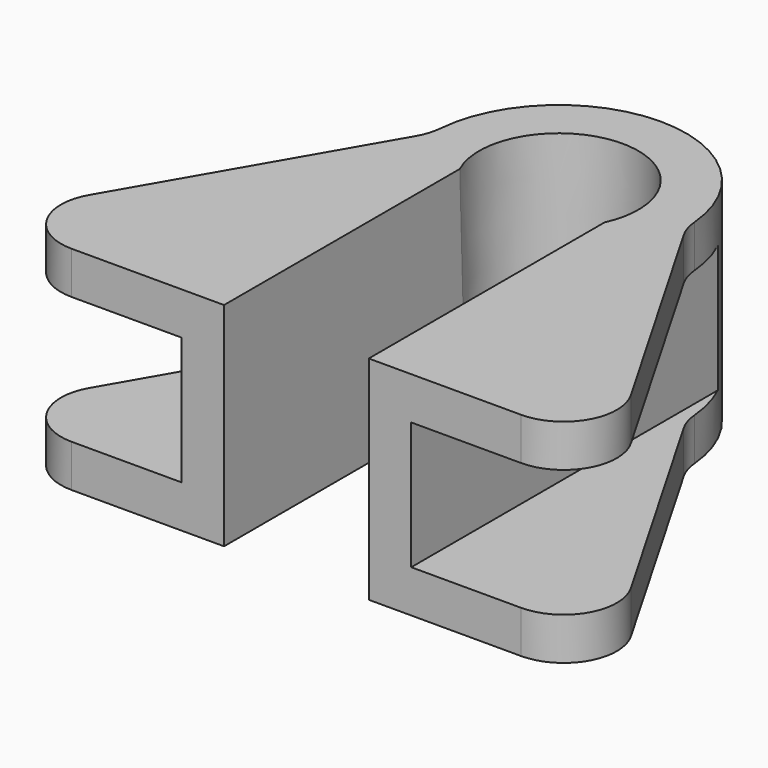
from build123d import *

# Parameters (mm, degrees)
F3_R      = 24
F4_DEPTH  = 40
F0_R      = 15
F2_R      = 14.5
F7_DEPTH  = 40.0010001
F9_DEPTH  = 40
F10_W     = 38.0299583572
F10_H     = 24
F11_DEPTH = 85.7581399225
F12_R     = 10
F13_R     = 10


# Not quite as in the source:
# - a pattern or mirror of a feature is missing from the dataset's text; its kind, count and spacing are read off the source's solid


with BuildPart() as f4:
    # F3 (on Top) → F4 (new body)
    with BuildSketch(Plane.XY):
        Circle(F3_R)
    extrude(amount=-F4_DEPTH)

    # F0 (on Top) → F5 section 0
    with BuildSketch(Plane.XY):
        Circle(F0_R)
    # F2 (on offset) → F5 section 1
    with BuildSketch(Plane.XY.offset(-40)):
        Circle(F2_R)
    loft(mode=Mode.SUBTRACT)

    # F6 (on face) → F7 (cut, through all)
    with BuildSketch(Plane.XY):
        with BuildLine():
            Line((-13.6255430014, -6.272525641), (-13.6255430014, -19.7571399225))
            ThreePointArc((-13.6255430014, -19.7571399225), (0, -24), (13.6255430014, -19.7571399225))
            Line((13.6255430014, -19.7571399225), (13.6255430014, -6.272525641))
            ThreePointArc((13.6255430014, -6.272525641), (0, -15), (-13.6255430014, -6.272525641))
        make_face()
        with BuildLine():
            Line((-13.6255430014, -4.9592920782), (-13.6255430014, -6.272525641))
            ThreePointArc((-13.6255430014, -6.272525641), (0, -15), (13.6255430014, -6.272525641))
            Line((13.6255430014, -6.272525641), (13.6255430014, -4.9592920782))
            ThreePointArc((13.6255430014, -4.9592920782), (0, -14.5), (-13.6255430014, -4.9592920782))
        make_face()
    extrude(amount=-F7_DEPTH, mode=Mode.SUBTRACT)

    # F8 (on face) → F9 (join)
    with BuildSketch(Plane.XY):
        with BuildLine():
            Line((-13.6255430014, -61.7571399225), (-13.6255430014, -19.7571399225))
            ThreePointArc((-13.6255430014, -19.7571399225), (-21.248682689, -11.1576648087), (-24, 0))
            Line((-24, 0), (-59.6555013586, -61.7571399225))
            Line((-59.6555013586, -61.7571399225), (-13.6255430014, -61.7571399225))
        make_face()
        with BuildLine():
            ThreePointArc((24, 0), (21.248682689, -11.1576648087), (13.6255430014, -19.7571399225))
            Line((13.6255430014, -19.7571399225), (13.6255430014, -61.7571399225))
            Line((13.6255430014, -61.7571399225), (59.6555013586, -61.7571399225))
            Line((59.6555013586, -61.7571399225), (24, 0))
        make_face()
    extrude(amount=-F9_DEPTH)

    # F10 (on face) → F11 (cut, through all)
    with BuildSketch(Plane.XZ.offset(61.7571399225)):
        with Locations((-40.64052218, -20)):
            Rectangle(F10_W, F10_H)
    f11 = extrude(amount=-F11_DEPTH, mode=Mode.SUBTRACT)

    # F11_copies: F11 across plane
    add(f11.mirror(Plane(origin=(0, 0, 0), x_dir=(0, 0, 1), z_dir=(1, 0, 0))), mode=Mode.SUBTRACT)

    # F12
    f12_edges = [f4.edges().sort_by_distance(p)[0] for p in [
        (-59.655501, -61.75714, -4),
        (-59.655501, -61.75714, -36),
        (-24, 0, -4),
        (-24, 0, -36),
    ]]
    fillet(f12_edges, radius=F12_R)

    # F13
    f13_edges = [f4.edges().sort_by_distance(p)[0] for p in [
        (59.655501, -61.75714, -4),
        (59.655501, -61.75714, -36),
        (24, 0, -4),
        (24, 0, -36),
    ]]
    fillet(f13_edges, radius=F13_R)


solid = f4.part
